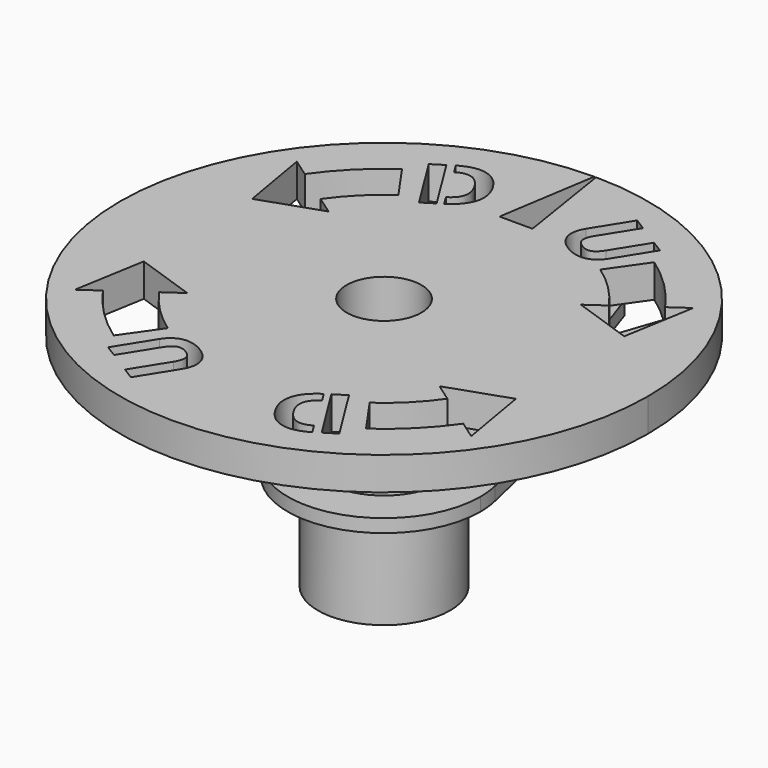
from build123d import *

# Parameters (mm, degrees)
F0_R         = 4.05
F0_R_2       = 3.4
F1_DEPTH     = 10
F2_R         = 24
F2_R_2       = 4.05
F2_R_3       = 3.4
F3_DEPTH     = 3
F4_TEXT_SIZE = 8.3333333333
F5_DEPTH     = 3
F5_FACE_W    = 0.5403645833
F5_FACE_H    = 3
F5_FACE1_W   = 0.6705729167
F5_FACE1_H   = 3
F5_FACE2_W   = 0.6705729167
F5_FACE2_H   = 3
F5_FACE3_W   = 0.5403645833
F5_FACE3_H   = 3
F10_R        = 6
F11_DEPTH    = 1.2
F10_R_2      = 5.28
F12_DEPTH    = 10


# Not quite as in the source:
# - Text() gives the source's letters only with a copy of the font that has no kerning and outlines rounded to 1/6400 em; it was checked with that copy


with BuildPart() as f1:
    # F0 (on Top) → F1 (new body)
    with BuildSketch(Plane.XY):
        Circle(F0_R)
        Circle(F0_R_2, mode=Mode.SUBTRACT)
    extrude(amount=F1_DEPTH)

    # F2 (on face) → F3 (join)
    with BuildSketch(Plane.XY.offset(10)):
        Circle(F2_R)
        Circle(F2_R_2, mode=Mode.SUBTRACT)
        Circle(F2_R_2)
        Circle(F2_R_3, mode=Mode.SUBTRACT)
    extrude(amount=F3_DEPTH)

    # F4 (on face) → F5 (cut, through all)
    with BuildSketch(Plane.XY.offset(13)):
        with BuildLine():
            ThreePointArc((0.0789678814, 23.9998700845), (0, 24), (-0.0789678814, 23.9998700845))
            Line((-0.0789678814, 23.9998700845), (-1.5, 15))
            Line((-1.5, 15), (0, 15))
            Line((0, 15), (1.5, 15))
            Line((1.5, 15), (0.0789678814, 23.9998700845))
        make_face()
        with BuildLine():
            Line((0.0789678814, 23.9998700845), (0, 24.5))
            Line((0, 24.5), (-0.0789678814, 23.9998700845))
            ThreePointArc((-0.0789678814, 23.9998700845), (0, 24), (0.0789678814, 23.9998700845))
        make_face()
        with BuildLine():
            Line((11.471528727, 16.3830408858), (10.3243758543, 14.7447367972))
            Line((10.3243758543, 14.7447367972), (9.1772229816, 13.1064327086))
            ThreePointArc((9.1772229816, 13.1064327086), (11.313708499, 11.313708499), (13.1064327086, 9.1772229816))
            Line((13.1064327086, 9.1772229816), (14.7447367972, 10.3243758543))
            Line((14.7447367972, 10.3243758543), (16.3830408858, 11.471528727))
            ThreePointArc((16.3830408858, 11.471528727), (14.1421356237, 14.1421356237), (11.471528727, 16.3830408858))
        make_face()
        Polygon((18.0213449744, 12.6186815997), (16.3830408858, 11.471528727), (14.7447367972, 10.3243758543), (13.1064327086, 9.1772229816), (11.46812862, 8.0300701089), (16.9144671741, 6.1563625799), align=None)
        with Locations(Location((2.7489732281, 15.969926931), (0, 0, -32))):
            Text('U', F4_TEXT_SIZE, font='Open Sans', font_style=FontStyle.BOLD, text_align=(TextAlign.LEFT, TextAlign.BOTTOM))
        with BuildLine():
            Line((-18.0213449744, 12.6186815997), (-16.9144671741, 6.1563625799))
            Line((-16.9144671741, 6.1563625799), (-11.46812862, 8.0300701089))
            Line((-11.46812862, 8.0300701089), (-13.1064327086, 9.1772229816))
            ThreePointArc((-13.1064327086, 9.1772229816), (-11.313708499, 11.313708499), (-9.1772229816, 13.1064327086))
            Line((-9.1772229816, 13.1064327086), (-10.3243758543, 14.7447367972))
            Line((-10.3243758543, 14.7447367972), (-11.471528727, 16.3830408858))
            ThreePointArc((-11.471528727, 16.3830408858), (-14.1421356237, 14.1421356237), (-16.3830408858, 11.471528727))
            Line((-16.3830408858, 11.471528727), (-18.0213449744, 12.6186815997))
        make_face()
        with BuildLine():
            Line((-11.471528727, -16.3830408858), (-10.3243758543, -14.7447367972))
            Line((-10.3243758543, -14.7447367972), (-9.1772229816, -13.1064327086))
            ThreePointArc((-9.1772229816, -13.1064327086), (-11.313708499, -11.313708499), (-13.1064327086, -9.1772229816))
            Line((-13.1064327086, -9.1772229816), (-11.46812862, -8.0300701089))
            Line((-11.46812862, -8.0300701089), (-16.9144671741, -6.1563625799))
            Line((-16.9144671741, -6.1563625799), (-18.0213449744, -12.6186815997))
            Line((-18.0213449744, -12.6186815997), (-16.3830408858, -11.471528727))
            ThreePointArc((-16.3830408858, -11.471528727), (-14.1421356237, -14.1421356237), (-11.471528727, -16.3830408858))
        make_face()
        with BuildLine():
            Line((16.9144671741, -6.1563625799), (11.46812862, -8.0300701089))
            Line((11.46812862, -8.0300701089), (13.1064327086, -9.1772229816))
            ThreePointArc((13.1064327086, -9.1772229816), (11.313708499, -11.313708499), (9.1772229816, -13.1064327086))
            Line((9.1772229816, -13.1064327086), (10.3243758543, -14.7447367972))
            Line((10.3243758543, -14.7447367972), (11.471528727, -16.3830408858))
            ThreePointArc((11.471528727, -16.3830408858), (14.1421356237, -14.1421356237), (16.3830408858, -11.471528727))
            Line((16.3830408858, -11.471528727), (18.0213449744, -12.6186815997))
            Line((18.0213449744, -12.6186815997), (16.9144671741, -6.1563625799))
        make_face()
        with Locations(Location((-7.9487889635, 12.7207214423), (0, 0, 32))):
            Text('D', F4_TEXT_SIZE, font='Open Sans', font_style=FontStyle.BOLD, text_align=(TextAlign.LEFT, TextAlign.BOTTOM))
        with Locations(Location((7.9487889635, -12.7207214423), (0, 0, -148))):
            Text('D', F4_TEXT_SIZE, font='Open Sans', font_style=FontStyle.BOLD, text_align=(TextAlign.LEFT, TextAlign.BOTTOM))
        with Locations(Location((-2.7489732281, -15.969926931), (0, 0, 148))):
            Text('U', F4_TEXT_SIZE, font='Open Sans', font_style=FontStyle.BOLD, text_align=(TextAlign.LEFT, TextAlign.BOTTOM))
    extrude(amount=-F5_DEPTH, mode=Mode.SUBTRACT)

    # F5_face (on face) → F6 (join, up to the next surface of F1)
    with BuildSketch(Plane(origin=(-6.5667305924, 14.8126381979, 11.5), x_dir=(0.8480480962, 0.5299192642, 0), z_dir=(0.5299192642, -0.8480480962, 0))):
        Rectangle(F5_FACE_W, F5_FACE_H)
    extrude(until=Until.NEXT)

    # F5_face1 (on face) → F7 (join, up to the next surface of F1)
    with BuildSketch(Plane(origin=(-8.5642662776, 18.1322202933, 11.5), x_dir=(-0.8480480962, -0.5299192642, 0), z_dir=(-0.5299192642, 0.8480480962, 0))):
        Rectangle(F5_FACE1_W, F5_FACE1_H)
    extrude(until=Until.NEXT)

    # F5_face2 (on face) → F8 (join, up to the next surface of F1)
    with BuildSketch(Plane(origin=(8.5642662776, -18.1322202933, 11.5), x_dir=(0.8480480962, 0.5299192642, 0), z_dir=(0.5299192642, -0.8480480962, 0))):
        Rectangle(F5_FACE2_W, F5_FACE2_H)
    extrude(until=Until.NEXT)

    # F5_face3 (on face) → F9 (join, up to the next surface of F1)
    with BuildSketch(Plane(origin=(6.5667305924, -14.8126381979, 11.5), x_dir=(-0.8480480962, -0.5299192642, 0), z_dir=(-0.5299192642, 0.8480480962, 0))):
        Rectangle(F5_FACE3_W, F5_FACE3_H)
    extrude(until=Until.NEXT)


with BuildPart() as f11:
    # F10 (on Top) → F11 (new body)
    with BuildSketch(Plane.XY):
        with BuildLine():
            ThreePointArc((-8.5271867369, 1.9620362774), (-0.9873236683, -8.6941182402), (8.75, 0))
            ThreePointArc((8.75, 0), (8.6941182402, 0.9873236683), (8.5271867369, 1.9620362774))
            ThreePointArc((8.5271867369, 1.9620362774), (0, 8.75), (-8.5271867369, 1.9620362774))
        make_face()
        Circle(F10_R, mode=Mode.SUBTRACT)
        with BuildLine():
            ThreePointArc((-8.5271867369, 1.9620362774), (0, 8.75), (8.5271867369, 1.9620362774))
            Line((8.5271867369, 1.9620362774), (2.0926942123, 29.9269215078))
            Line((2.0926942123, 29.9269215078), (0.0789678814, 23.9998700845))
            Line((0.0789678814, 23.9998700845), (-0.0789678814, 23.9998700845))
            Line((-0.0789678814, 23.9998700845), (-2.0926942123, 29.9269215078))
            Line((-2.0926942123, 29.9269215078), (-8.5271867369, 1.9620362774))
        make_face()
    extrude(amount=-F11_DEPTH)

    # F10 (on Top) → F12 (join)
    with BuildSketch(Plane.XY):
        Circle(F10_R)
        Circle(F10_R_2, mode=Mode.SUBTRACT)
    extrude(amount=-F12_DEPTH)


solid = Compound([f1.part, f11.part])
